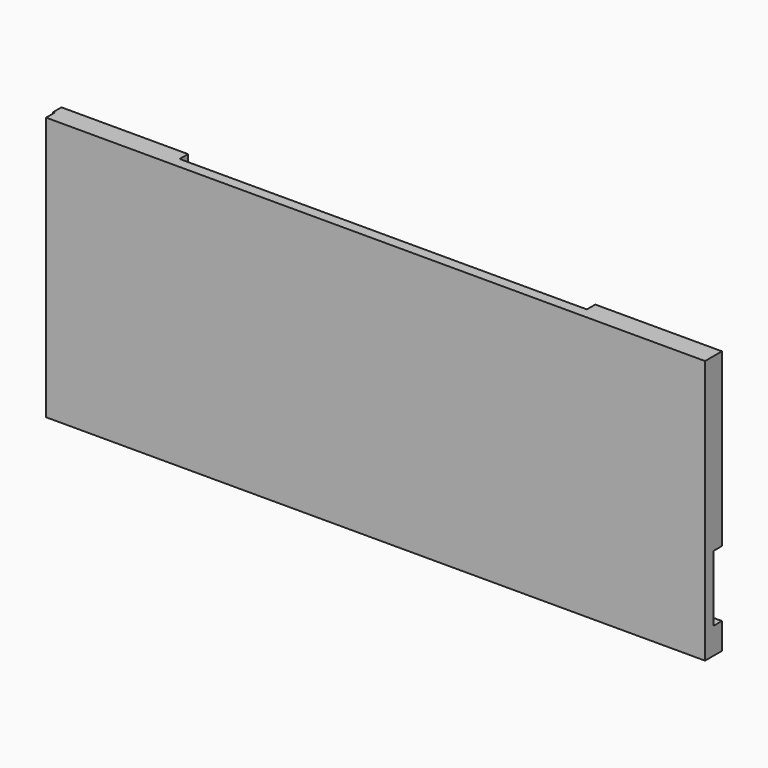
from build123d import *

# Parameters (mm, degrees)
F0_W      = 249.8
F0_H      = 100
F1_DEPTH  = 4
F4_W      = 20
F4_H      = 10
F5_DEPTH  = 4
F6_W      = 48
F6_H      = 65
F7_DEPTH  = 4
F8_W      = 20
F8_H      = 10
F9_DEPTH  = 4
F10_DEPTH = 1.1
F11_W     = 20
F11_H     = 3.2
F12_DEPTH = 13
F13_SIZE  = 12.1
F14_R     = 2


# Not quite as in the source:
# - a feature names something its author has since deleted; it is built from what else it names


with BuildPart() as f1:
    # F0 (on Front) → F1 (new body)
    with BuildSketch(Plane.XZ):
        with Locations((0.2878084779, -20.9680776408)):
            Rectangle(F0_W, F0_H)
    extrude(amount=F1_DEPTH)

    # F4 (on face) → F5 (join)
    with BuildSketch(Plane(origin=(0, 0, 0), x_dir=(-1, 0, 0), z_dir=(0, 1, 0))):
        with Locations((-115.1878084779, -65.9680776408)):
            Rectangle(F4_W, F4_H)
        with Locations((114.6121915221, -65.9680776408)):
            Rectangle(F4_W, F4_H)
    extrude(amount=F5_DEPTH)

    # F6 (on face) → F7 (join)
    with BuildSketch(Plane(origin=(0, 0, 0), x_dir=(-1, 0, 0), z_dir=(0, 1, 0))):
        with Locations((-101.1878084779, -3.4680776408)):
            Rectangle(F6_W, F6_H)
        with Locations((101.1878084779, -3.4680776408)):
            Rectangle(F6_W, F6_H)
    extrude(amount=F7_DEPTH)

    # F8 (on face) → F9 (join)
    with BuildSketch(Plane(origin=(0, 0, 0), x_dir=(-1, 0, 0), z_dir=(0, 1, 0))):
        with Locations((114.6121915221, -65.9680776408)):
            Rectangle(F8_W, F8_H)
    extrude(amount=F9_DEPTH)

    # F2 (on face) → F10 (cut)
    with BuildSketch(Plane(origin=(0, 0, 0), x_dir=(-1, 0, 0), z_dir=(0, 1, 0))):
        Polygon((41.6121915221, 16.0319223592), (-44.3878084779, 16.0319223592), (-44.3878084779, 6.0319223592), (-44.3878084779, -23.9680776408), (-44.3878084779, -33.9680776408), (41.6121915221, -33.9680776408), (41.6121915221, 6.0319223592), align=None)
    extrude(amount=-F10_DEPTH, mode=Mode.SUBTRACT)

    # F11 (on face) → F12 (join)
    with BuildSketch(Plane(origin=(0, 4, 0), x_dir=(-1, 0, 0), z_dir=(0, 1, 0))):
        with Locations((-97.1878084779, -26.3680776408)):
            Rectangle(F11_W, F11_H)
        with Locations((97.1878084779, -26.3680776408)):
            Rectangle(F11_W, F11_H)
    extrude(amount=F12_DEPTH)

    # F13
    f13_edges = [f1.edges().sort_by_distance(p)[0] for p in [
        (87.187808, 17, -26.368078),
        (-87.187808, 17, -26.368078),
    ]]
    chamfer(f13_edges, length=F13_SIZE)

    # F14
    f14_edges = [f1.edges().sort_by_distance(p)[0] for p in [
        (107.187808, 17, -26.368078),
        (-107.187808, 17, -26.368078),
    ]]
    fillet(f14_edges, radius=F14_R)


solid = f1.part
